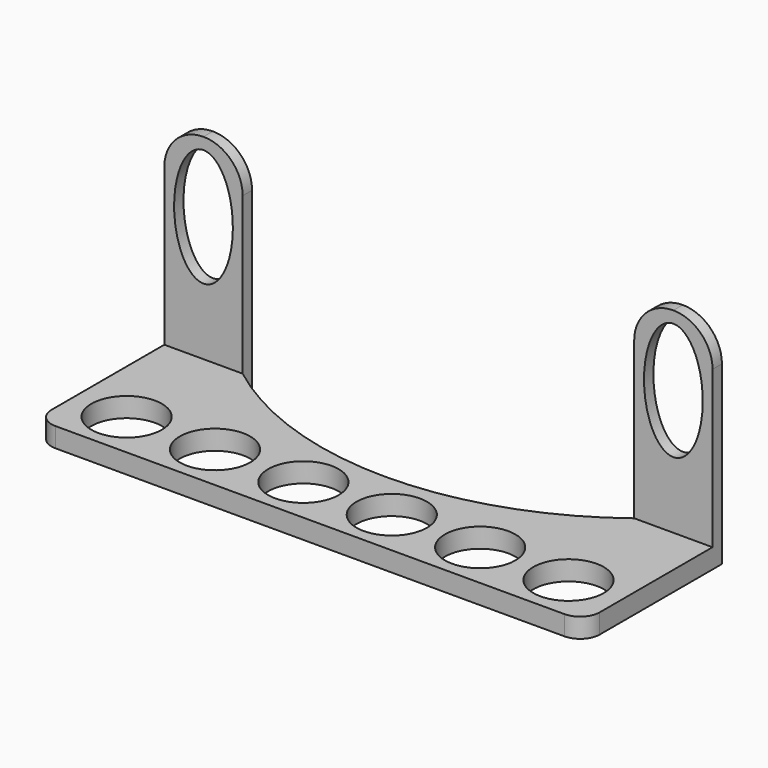
from build123d import *

# Parameters (mm, degrees)
F0_R     = 9
F0_W     = 20
F0_H     = 3
F1_DEPTH = 5
F2_DEPTH = 50
F4_DEPTH = 12.5
F5_R     = 9.99999


# Not quite as in the source:
# - a fillet or chamfer is up to 0.001 mm smaller than in the source, because OpenCascade refuses the exact size


with BuildPart() as f1:
    # F0 (on Top) → F1 (new body)
    with BuildSketch(Plane.XY):
        with BuildLine():
            Line((-70, -3), (-70, -20))
            Line((-70, -20), (2.765e-07, -20))
            ThreePointArc((2.765e-07, -20), (-26.4054917221, -15.6337996122), (-50, -3))
            Line((-50, -3), (-70, -3))
        make_face()
        with BuildLine():
            Line((2.765e-07, -20), (-70, -20))
            Line((-70, -20), (-70, -39))
            ThreePointArc((-70, -39), (-68.5355339059, -42.5355339059), (-65, -44))
            Line((-65, -44), (65, -44))
            ThreePointArc((65, -44), (68.5355339059, -42.5355339059), (70, -39))
            Line((70, -39), (70, -20))
            Line((70, -20), (2.765e-07, -20))
        make_face()
        with Locations((-56.4285714286, -32)):
            Circle(F0_R, mode=Mode.SUBTRACT)
        with Locations((-33.8571428571, -32)):
            Circle(F0_R, mode=Mode.SUBTRACT)
        with Locations((-11.2857142857, -32)):
            Circle(F0_R, mode=Mode.SUBTRACT)
        with Locations((11.2857142857, -32)):
            Circle(F0_R, mode=Mode.SUBTRACT)
        with Locations((33.8571428571, -32)):
            Circle(F0_R, mode=Mode.SUBTRACT)
        with Locations((56.4285714286, -32)):
            Circle(F0_R, mode=Mode.SUBTRACT)
        with BuildLine():
            ThreePointArc((50, -3), (26.4054919839, -15.6337995232), (2.765e-07, -20))
            Line((2.765e-07, -20), (70, -20))
            Line((70, -20), (70, -3))
            Line((70, -3), (50, -3))
        make_face()
        with Locations((-60, -1.5)):
            Rectangle(F0_W, F0_H)
        with Locations((60, -1.5)):
            Rectangle(F0_W, F0_H)
    extrude(amount=-F1_DEPTH)

    # F0 (on Top) → F2 (join)
    with BuildSketch(Plane.XY):
        with Locations((-60, -1.5)):
            Rectangle(F0_W, F0_H)
        with Locations((60, -1.5)):
            Rectangle(F0_W, F0_H)
    extrude(amount=F2_DEPTH)

    # F3 (on face) → F4 (cut, symmetric)
    with BuildSketch(Plane.XZ.offset(3)):
        with BuildLine():
            add(Edge.make_bspline(
                [(-60, 17), (-47.0096189432, 17), (-53.5048094716, 39.5), (-60, 62), (-66.4951905284, 39.5), (-72.9903810568, 17), (-60, 17)],
                knots=[0, 0, 0, 2.0943951024, 2.0943951024, 4.1887902048, 4.1887902048, 6.2831853072, 6.2831853072, 6.2831853072], degree=2, weights=[1, 0.5, 1, 0.5, 1, 0.5, 1]))
        make_face()
        with BuildLine():
            add(Edge.make_bspline(
                [(60, 17), (72.9903810568, 17), (66.4951905284, 39.5), (60, 62), (53.5048094716, 39.5), (47.0096189432, 17), (60, 17)],
                knots=[0, 0, 0, 2.0943951024, 2.0943951024, 4.1887902048, 4.1887902048, 6.2831853072, 6.2831853072, 6.2831853072], degree=2, weights=[1, 0.5, 1, 0.5, 1, 0.5, 1]))
        make_face()
    extrude(amount=F4_DEPTH, both=True, mode=Mode.SUBTRACT)

    # F5 (radius 10 in the source; OpenCascade refuses exactly that, so slightly less here)
    f5_edges = [f1.edges().sort_by_distance(p)[0] for p in [
        (-70, -1.5, 50),
        (-50, -1.5, 50),
        (70, -1.5, 50),
        (50, -1.5, 50),
    ]]
    fillet(f5_edges, radius=F5_R)


solid = f1.part
